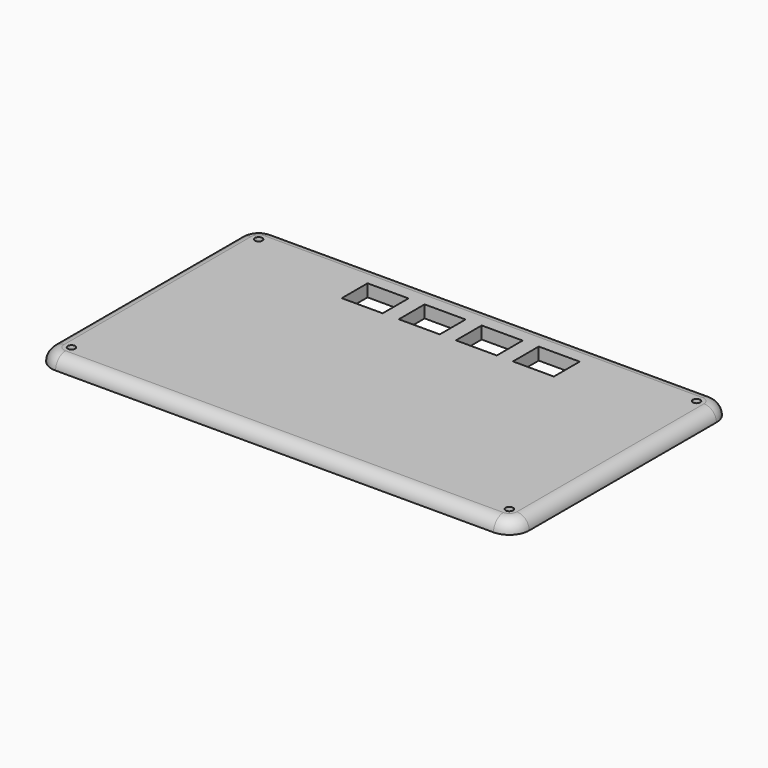
from build123d import *

# Parameters (mm, degrees)
F1_DEPTH = 5
F2_R     = 1.5
F3_DEPTH = 5.001
F4_DEPTH = 25
F5_R     = 4.99999
F6_W     = 16.5
F6_H     = 13
F7_DEPTH = 5.001
F9_DEPTH = 1.5


# Not quite as in the source:
# - a fillet or chamfer is up to 0.001 mm smaller than in the source, because OpenCascade refuses the exact size


with BuildPart() as f1:
    # F0 (on Top) → F1 (new body)
    with BuildSketch(Plane.XY):
        with BuildLine():
            ThreePointArc((-61.6726832837, -15.8819631437), (-59.3295375332, -21.5388173932), (-53.6726832837, -23.8819631437))
            Line((-53.6726832837, -23.8819631437), (122.8273167163, -23.8819631437))
            ThreePointArc((122.8273167163, -23.8819631437), (128.4841709658, -21.5388173932), (130.8273167163, -15.8819631437))
            Line((130.8273167163, -15.8819631437), (130.8273167163, 78.4180368563))
            ThreePointArc((130.8273167163, 78.4180368563), (128.4841709658, 84.0748911058), (122.8273167163, 86.4180368563))
            Line((122.8273167163, 86.4180368563), (-53.6726832837, 86.4180368563))
            ThreePointArc((-53.6726832837, 86.4180368563), (-59.3295375332, 84.0748911058), (-61.6726832837, 78.4180368563))
            Line((-61.6726832837, 78.4180368563), (-61.6726832837, -15.8819631437))
        make_face()
    extrude(amount=-F1_DEPTH)

    # F2 (on face) → F3 (cut, through all)
    with BuildSketch(Plane(origin=(0, 0, -5), x_dir=(1, 0, 0), z_dir=(0, 0, -1))):
        with Locations((-53.6726832837, 15.8819631437)):
            Circle(F2_R)
        with Locations((122.8273167163, 15.8819631437)):
            Circle(F2_R)
        with Locations((122.8273167163, -78.4180368563)):
            Circle(F2_R)
        with Locations((-53.6726832837, -78.4180368563)):
            Circle(F2_R)
    extrude(amount=-F3_DEPTH, mode=Mode.SUBTRACT)

    # F4 (cut): a face of the model
    f4_faces = [f1.faces().sort_by_distance(p)[0] for p in [
        (34.5773167163, 31.2680368563, -5),
    ]]
    extrude(f4_faces, amount=F4_DEPTH, mode=Mode.SUBTRACT)

    # F5 (radius 5 in the source; OpenCascade refuses exactly that, so slightly less here)
    f5_edges = [f1.edges().sort_by_distance(p)[0] for p in [
        (34.577317, 86.418037, 0),
        (128.484171, 84.074891, 0),
        (130.827317, 31.268037, 0),
        (128.484171, -21.538817, 0),
        (34.577317, -23.881963, 0),
        (-59.329538, -21.538817, 0),
        (-61.672683, 31.268037, 0),
        (-59.329538, 84.074891, 0),
    ]]
    fillet(f5_edges, radius=F5_R)

    # F6 (on face) → F7 (cut, through all)
    with BuildSketch(Plane.XY):
        with Locations((0.0773167163, 69.9180368563)):
            Rectangle(F6_W, F6_H)
        with Locations((23.0773167163, 69.9180368563)):
            Rectangle(F6_W, F6_H)
        with Locations((46.0773167163, 69.9180368563)):
            Rectangle(F6_W, F6_H)
        with Locations((69.0773167163, 69.9180368563)):
            Rectangle(F6_W, F6_H)
    extrude(amount=-F7_DEPTH, mode=Mode.SUBTRACT)

    # F8 (on face) → F9 (cut)
    with BuildSketch(Plane(origin=(0, 0, -5), x_dir=(1, 0, 0), z_dir=(0, 0, -1))):
        Polygon((-43.6726832837, -69.9180368563), (-46.6726832837, -69.9180368563), (-46.6726832837, -80.4180368563), (-36.1726832837, -80.4180368563), (-36.1726832837, -77.4180368563), (-43.6726832837, -77.4180368563), align=None)
        Polygon((-46.6726832837, 7.3819631437), (-43.6726832837, 7.3819631437), (-43.6726832837, 14.8819631437), (-36.1726832837, 14.8819631437), (-36.1726832837, 17.8819631437), (-46.6726832837, 17.8819631437), align=None)
        Polygon((115.8273167163, 17.8819631437), (105.3273167163, 17.8819631437), (105.3273167163, 14.8819631437), (112.8273167163, 14.8819631437), (112.8273167163, 7.3819631437), (115.8273167163, 7.3819631437), align=None)
        Polygon((115.8273167163, -69.9180368563), (112.8273167163, -69.9180368563), (112.8273167163, -77.4180368563), (105.3273167163, -77.4180368563), (105.3273167163, -80.4180368563), (115.8273167163, -80.4180368563), align=None)
    extrude(amount=-F9_DEPTH, mode=Mode.SUBTRACT)


solid = f1.part
